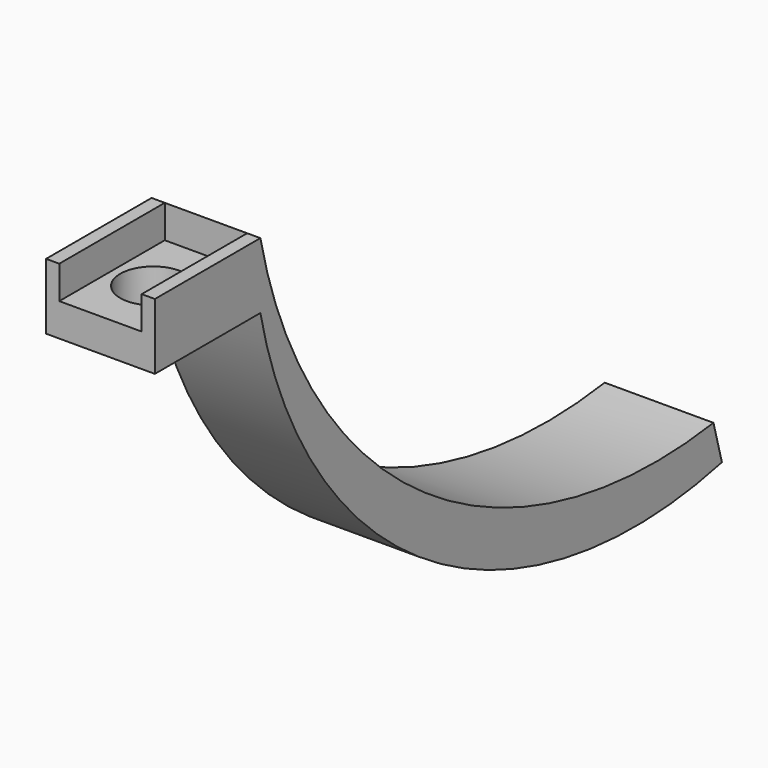
from build123d import *

# Parameters (mm, degrees)
F1_DEPTH = 2.0955
F2_R     = 0.635
F3_DEPTH = 25.4
F4_W     = 1.5875
F4_H     = 2.5404572
F4_R     = 0.635
F5_DEPTH = 0.635


# Not quite as in the source:
# - a feature names something its author has since deleted; it is built from what else it names


with BuildPart() as f1:
    # F0 (on Right) → F1 (new body)
    with BuildSketch(Plane.YZ):
        with BuildLine():
            Line((51.3955118105, -18.3105177657), (51.3955118105, -19.5805177657))
            Line((51.3955118105, -19.5805177657), (53.9359690105, -19.5805177657))
            ThreePointArc((53.9359690105, -19.5805177657), (58.0135640106, -25.4388820379), (65.0510564446, -26.6309026629))
            Line((65.0510564446, -26.6309026629), (64.8478195071, -25.8786771446))
            ThreePointArc((64.8478195071, -25.8786771446), (57.9021718289, -24.2424946681), (53.9359690105, -18.3105177657))
            Line((53.9359690105, -18.3105177657), (51.3955118105, -18.3105177657))
        make_face()
    extrude(amount=F1_DEPTH)

    # F2 (on face) → F3 (cut)
    with BuildSketch(Plane(origin=(0, 0, -19.5805177657), x_dir=(1, 0, 0), z_dir=(0, 0, -1))):
        with Locations((1.04775, -52.6657345776)):
            Circle(F2_R)
    extrude(amount=-F3_DEPTH, mode=Mode.SUBTRACT)

    # F4 (on face) → F5 (cut)
    with BuildSketch(Plane.XY.offset(-18.3105177657)):
        with Locations((1.04775, 52.6657404105)):
            Rectangle(F4_W, F4_H)
        with Locations((1.04775, 52.6657345776)):
            Circle(F4_R, mode=Mode.SUBTRACT)
    extrude(amount=-F5_DEPTH, mode=Mode.SUBTRACT)


solid = f1.part
